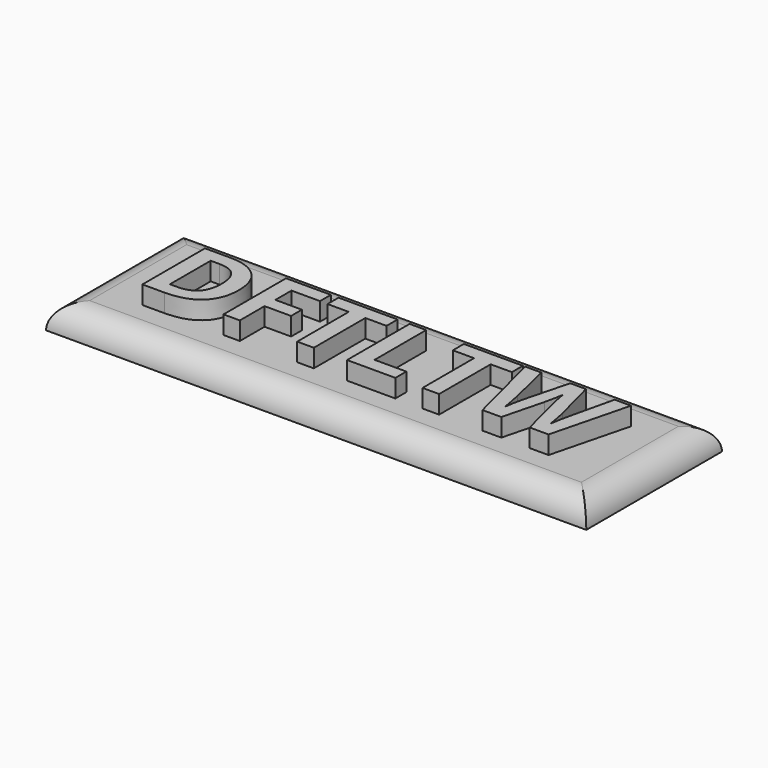
from build123d import *

# Parameters (mm, degrees)
F0_TEXT_SIZE = 22.9913796324
F1_DEPTH     = 3.81
F2_W         = 113.3844032884
F2_H         = 35.5899017304
F3_DEPTH     = 5.08
F4_R         = 5.07999
F5_TEXT_SIZE = 7.8529017196
F7_DEPTH     = 3.81
F6_TEXT_SIZE = 10.8382360648
F8_DEPTH     = 3.81


# Not quite as in the source:
# - a fillet or chamfer is up to 0.001 mm smaller than in the source, because OpenCascade refuses the exact size
# - Text() gives the source's letters only with a copy of the font that has no kerning and outlines rounded to 1/6400 em; it was checked with that copy


with BuildPart() as f1:
    # F0 (on Top) → F1 (new body)
    with BuildSketch(Plane.XY):
        with Locations((-46.7053465545, -7.4229317252)):
            Text('DFTLTW', F0_TEXT_SIZE, font='Open Sans', font_style=FontStyle.BOLD, text_align=(TextAlign.LEFT, TextAlign.BOTTOM))
    extrude(amount=F1_DEPTH)


with BuildPart() as f3:
    # F2 (on Top) → F3 (new body)
    with BuildSketch(Plane.XY):
        with Locations((-0.7633902133, 1.1167237535)):
            Rectangle(F2_W, F2_H)
    extrude(amount=-F3_DEPTH)

    # F4 (radius 5.08 in the source; OpenCascade refuses exactly that, so slightly less here)
    f4_edges = [f3.edges().sort_by_distance(p)[0] for p in [
        (-0.76339, 18.911675, 0),
        (-57.455592, 1.116724, 0),
        (-0.76339, -16.678227, 0),
        (55.928811, 1.116724, 0),
    ]]
    fillet(f4_edges, radius=F4_R)

    # F5 (on face) → F7 (cut)
    with BuildSketch(Plane(origin=(0, 0, -5.08), x_dir=(1, 0, 0), z_dir=(0, 0, -1))):
        with Locations((-45.4023323979, 3.9013231295)):
            Text('Love you more, and more', F5_TEXT_SIZE, font='Open Sans', text_align=(TextAlign.LEFT, TextAlign.BOTTOM))
    extrude(amount=-F7_DEPTH, mode=Mode.SUBTRACT)

    # F6 (on face) + F5 (on face) → F8 (cut)
    with BuildSketch(Plane(origin=(0, 0, -5.08), x_dir=(1, 0, 0), z_dir=(0, 0, -1))):
        with Locations((-49.5956912637, -13.406932354)):
            Text('every day!     - wifey', F6_TEXT_SIZE, font='Open Sans', text_align=(TextAlign.LEFT, TextAlign.BOTTOM))
    with BuildSketch(Plane(origin=(0, 0, -5.08), x_dir=(1, 0, 0), z_dir=(0, 0, -1))):
        with Locations((-45.4023323979, 3.9013231295)):
            Text('Love you more, and more', F5_TEXT_SIZE, font='Open Sans', text_align=(TextAlign.LEFT, TextAlign.BOTTOM))
    extrude(amount=-F8_DEPTH, mode=Mode.SUBTRACT)


solid = Compound([f1.part, f3.part])
